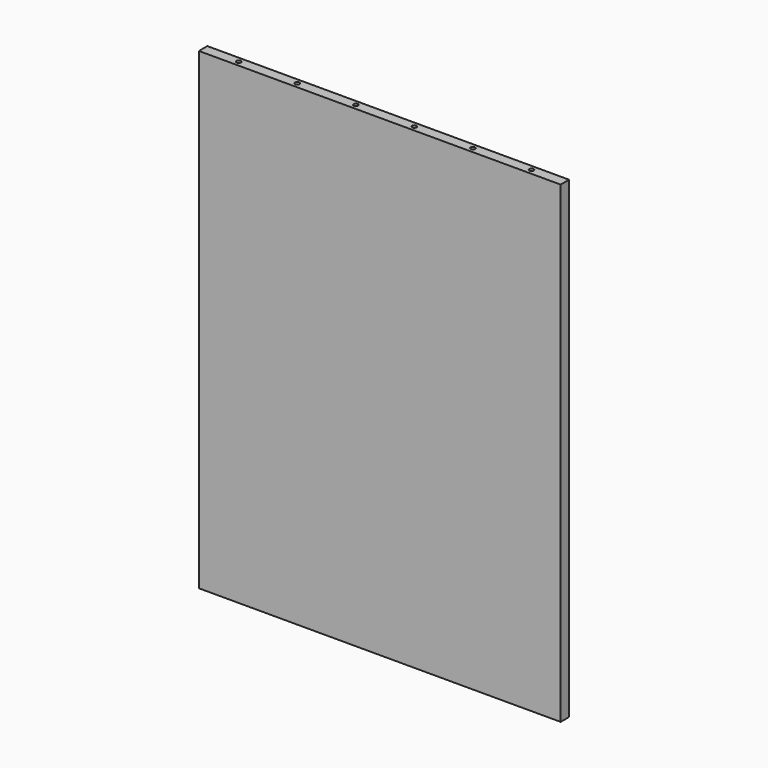
from build123d import *

# Parameters (mm, degrees)
F0_W     = 650
F0_H     = 850
F1_DEPTH = 19
F2_R     = 4
F3_DEPTH = 20


# Not quite as in the source:
# - a pattern or mirror of a feature is missing from the dataset's text; its kind, count and spacing are read off the source's solid


with BuildPart() as f1:
    # F0 (on Front) → F1 (new body)
    with BuildSketch(Plane.XZ):
        Rectangle(F0_W, F0_H)
    extrude(amount=F1_DEPTH)

    # F2 (on face) → F3 (cut)
    with BuildSketch(Plane.XY.offset(425)):
        with Locations((265, -9.5)):
            Circle(F2_R)
        with Locations((159.8, -9.5)):
            Circle(F2_R)
        with Locations((54.6, -9.5)):
            Circle(F2_R)
        with Locations((-50.6, -9.5)):
            Circle(F2_R)
        with Locations((-155.8, -9.5)):
            Circle(F2_R)
        with Locations((-261, -9.5)):
            Circle(F2_R)
    f3 = extrude(amount=-F3_DEPTH, mode=Mode.SUBTRACT)

    # F3_copies: F3 across plane
    add(f3.mirror(Plane(origin=(0, 0, 0), x_dir=(-1, 0, 0), z_dir=(0, 0, -1))), mode=Mode.SUBTRACT)


solid = f1.part
